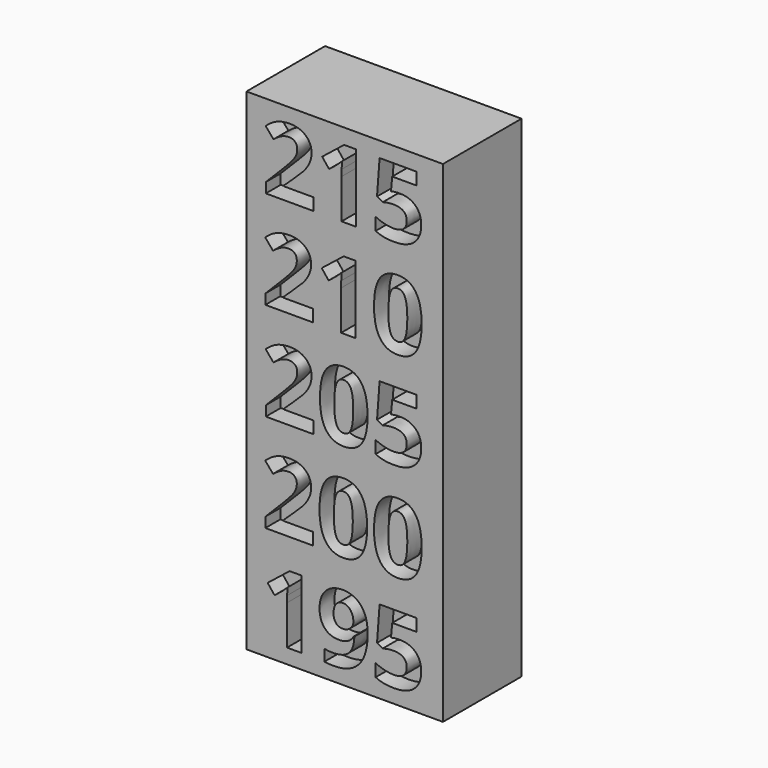
from build123d import *

# Parameters (mm, degrees)
F0_W         = 20
F0_H         = 10
F1_DEPTH     = 50
F2_TEXT_SIZE = 9.7222222222
F3_DEPTH     = 1.9


# Not quite as in the source:
# - Text() gives the source's letters only with a copy of the font that has no kerning and outlines rounded to 1/6400 em; it was checked with that copy


with BuildPart() as f1:
    # F0 (on Top) → F1 (new body)
    with BuildSketch(Plane.XY):
        Rectangle(F0_W, F0_H)
    extrude(amount=F1_DEPTH)

    # F2 (on face) → F3 (cut)
    with BuildSketch(Plane.XZ.offset(5)):
        with Locations((-8.4211154514, 41.5)):
            Text('215', F2_TEXT_SIZE, font='Open Sans', font_style=FontStyle.BOLD, text_align=(TextAlign.LEFT, TextAlign.BOTTOM))
        with Locations((-8.4659288194, 31.5)):
            Text('210', F2_TEXT_SIZE, font='Open Sans', font_style=FontStyle.BOLD, text_align=(TextAlign.LEFT, TextAlign.BOTTOM))
        with Locations((-8.4211154514, 21.5)):
            Text('205', F2_TEXT_SIZE, font='Open Sans', font_style=FontStyle.BOLD, text_align=(TextAlign.LEFT, TextAlign.BOTTOM))
        with Locations((-8.4659288194, 11.5)):
            Text('200', F2_TEXT_SIZE, font='Open Sans', font_style=FontStyle.BOLD, text_align=(TextAlign.LEFT, TextAlign.BOTTOM))
        with Locations((-8.4211154514, 1.5)):
            Text('195', F2_TEXT_SIZE, font='Open Sans', font_style=FontStyle.BOLD, text_align=(TextAlign.LEFT, TextAlign.BOTTOM))
    extrude(amount=-F3_DEPTH, mode=Mode.SUBTRACT)


solid = f1.part
